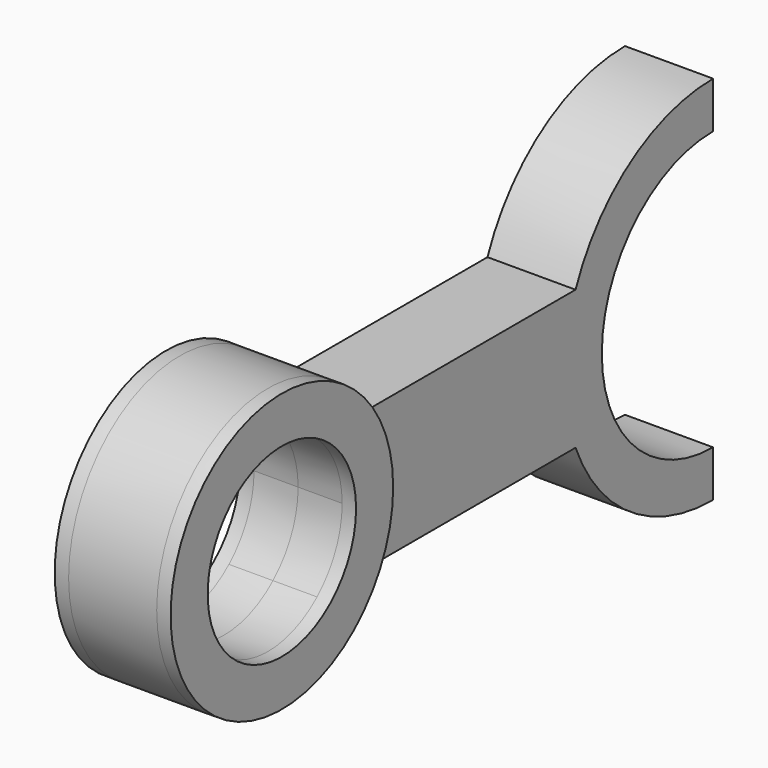
from build123d import *
from build123d import SkipClean  # not in build123d's __all__

# Parameters (mm, degrees)
F1_DEPTH = 12.065
F2_R     = 38.1
F2_R_2   = 25.4
F3_DEPTH = 15.875


with BuildPart() as f1:
    # F0 (on Right) → F1 (new body, symmetric)
    with BuildSketch(Plane.YZ):
        with BuildLine():
            ThreePointArc((39.5052965482, -19.05), (34.4008644324, 0), (39.5052965482, 19.05))
            Line((39.5052965482, 19.05), (25.4080040394, 19.05))
            ThreePointArc((25.4080040394, 19.05), (21.7008644324, 0), (25.4080040394, -19.05))
            Line((25.4080040394, -19.05), (39.5052965482, -19.05))
        make_face()
        with BuildLine():
            Line((25.4080040394, 19.05), (39.5052965482, 19.05))
            ThreePointArc((39.5052965482, 19.05), (53.4508644324, 32.9955678842), (72.5008644324, 38.1))
            Line((72.5008644324, 38.1), (72.5008644324, 50.8))
            ThreePointArc((72.5008644324, 50.8), (44.1028011182, 42.1211348375), (25.4080040394, 19.05))
        make_face()
        with BuildLine():
            ThreePointArc((25.4080040394, -19.05), (21.7008644324, 0), (25.4080040394, 19.05))
            Line((25.4080040394, 19.05), (-46.9035676834, 19.05))
            ThreePointArc((-46.9035676834, 19.05), (-43.097361586, 9.8610056184), (-41.7991355676, 0))
            ThreePointArc((-41.7991355676, 0), (-43.097361586, -9.8610056184), (-46.9035676834, -19.05))
            Line((-46.9035676834, -19.05), (25.4080040394, -19.05))
        make_face()
        with BuildLine():
            ThreePointArc((72.5008644324, -38.1), (53.4508644324, -32.9955678842), (39.5052965482, -19.05))
            Line((39.5052965482, -19.05), (25.4080040394, -19.05))
            ThreePointArc((25.4080040394, -19.05), (44.1028011182, -42.1211348375), (72.5008644324, -50.8))
            Line((72.5008644324, -50.8), (72.5008644324, -38.1))
        make_face()
        with BuildLine():
            ThreePointArc((-41.7991355676, 0), (-43.097361586, 9.8610056184), (-46.9035676834, 19.05))
            Line((-46.9035676834, 19.05), (-63.0986147423, 19.05))
            ThreePointArc((-63.0986147423, 19.05), (-56.7486147423, 10.4505208253), (-54.4991355676, 0))
            ThreePointArc((-54.4991355676, 0), (-56.7486147423, -10.4505208253), (-63.0986147423, -19.05))
            Line((-63.0986147423, -19.05), (-46.9035676834, -19.05))
            ThreePointArc((-46.9035676834, -19.05), (-43.097361586, -9.8610056184), (-41.7991355676, 0))
        make_face()
        with BuildLine():
            Line((-63.0986147423, 19.05), (-46.9035676834, 19.05))
            ThreePointArc((-46.9035676834, 19.05), (-117.9991355676, 0), (-46.9035676834, -19.05))
            Line((-46.9035676834, -19.05), (-63.0986147423, -19.05))
            ThreePointArc((-63.0986147423, -19.05), (-105.2991355676, 0), (-63.0986147423, 19.05))
        make_face()
    extrude(amount=F1_DEPTH, both=True)

    # F2 (on Right) → F3 (join, symmetric)
    with BuildSketch(Plane.YZ):
        with Locations((-79.8991355676, 0)):
            Circle(F2_R)
        with Locations((-79.8991355676, 0)):
            Circle(F2_R_2, mode=Mode.SUBTRACT)
    with SkipClean():  # cleaning this boolean's faces spoils the solid; the shape is the same uncleaned
        extrude(amount=F3_DEPTH, both=True)


solid = f1.part
